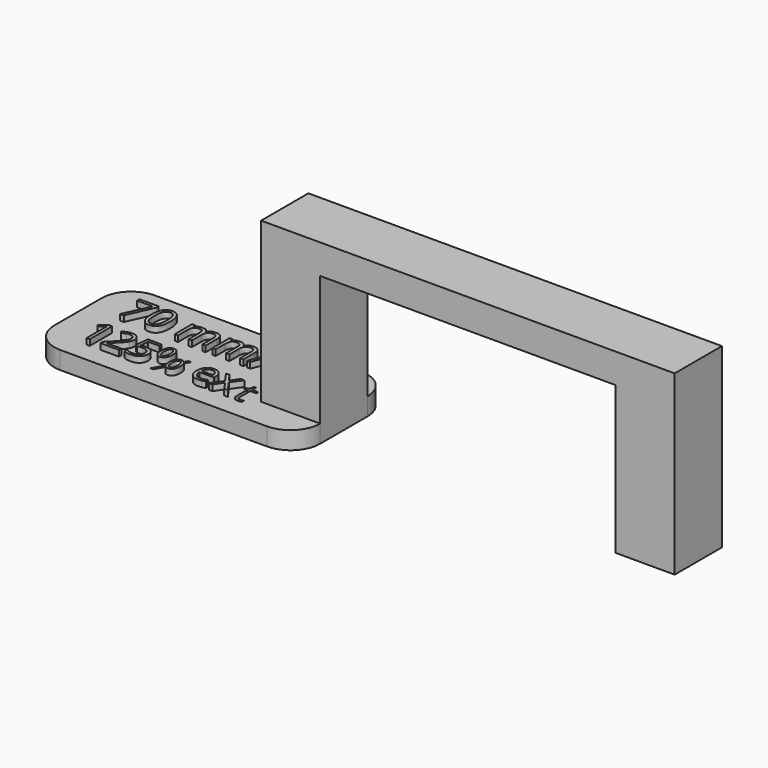
from build123d import *

# Parameters (mm, degrees)
F0_W         = 10
F0_H         = 10
F1_DEPTH     = 25
F2_START     = 25
F0_W_2       = 50
F2_DEPTH     = 5
F0_TEXT_SIZE = 6.8483603532
F3_DEPTH     = 3
F4_DEPTH     = 4


# Not quite as in the source:
# - Text() gives the source's letters only with a copy of the font that has no kerning and outlines rounded to 1/6400 em; it was checked with that copy


with BuildPart() as f1:
    # F0 (on Top) → F1 (new body)
    with BuildSketch(Plane.XY):
        with Locations((30, 0)):
            Rectangle(F0_W, F0_H)
    extrude(amount=F1_DEPTH)



with BuildPart() as f1b:
    # F0 (on Top) → F1, piece 2 (new body)
    with BuildSketch(Plane.XY):
        with Locations((-30, 0)):
            Rectangle(F0_W, F0_H)
    extrude(amount=F1_DEPTH)


with BuildPart() as f1_1:
    add(f1.part)

    add(f1b.part)  # F2 merges F1b
    # F0 (on Top) → F2 (join)
    with BuildSketch(Plane.XY.offset(F2_START)):
        Rectangle(F0_W_2, F0_H)
        with Locations((-30, 0)):
            Rectangle(F0_W, F0_H)
        with Locations((30, 0)):
            Rectangle(F0_W, F0_H)
    extrude(amount=F2_DEPTH)

    # F0 (on Top) → F3 (join)
    with BuildSketch(Plane.XY):
        with BuildLine():
            ThreePointArc((-30, -10), (-26.4644660941, -8.5355339059), (-25, -5))
            Line((-25, -5), (-35, -5))
            Line((-35, -5), (-35, 5))
            Line((-35, 5), (-25, 5))
            ThreePointArc((-25, 5), (-26.4644660941, 8.5355339059), (-30, 10))
            Line((-30, 10), (-65, 10))
            ThreePointArc((-65, 10), (-68.5355339059, 8.5355339059), (-70, 5))
            Line((-70, 5), (-70, -5))
            ThreePointArc((-70, -5), (-68.5355339059, -8.5355339059), (-65, -10))
            Line((-65, -10), (-30, -10))
        make_face()
        with BuildLine():
            add(Edge.make_bspline(
                [(-48.7220816963, -4.113544751), (-48.4639328914, -4.4947946962), (-48.4639328914, -5.2157414592)],
                knots=[0, 0, 0, 1, 1, 1], degree=2))
            add(Edge.make_bspline(
                [(-48.4639328914, -5.2157414592), (-48.4639328914, -5.9522706451), (-48.7122128285, -6.3309235199)],
                knots=[0, 0, 0, 1, 1, 1], degree=2))
            add(Edge.make_bspline(
                [(-48.7122128285, -6.3309235199), (-48.9604927656, -6.7095763947), (-49.441470217, -6.7095763947)],
                knots=[0, 0, 0, 1, 1, 1], degree=2))
            add(Edge.make_bspline(
                [(-49.441470217, -6.7095763947), (-49.9027099328, -6.7095763947), (-50.1509898699, -6.3231323084)],
                knots=[0, 0, 0, 1, 1, 1], degree=2))
            add(Edge.make_bspline(
                [(-50.1509898699, -6.3231323084), (-50.399269807, -5.9366882222), (-50.399269807, -5.2157414592)],
                knots=[0, 0, 0, 1, 1, 1], degree=2))
            add(Edge.make_bspline(
                [(-50.399269807, -5.2157414592), (-50.399269807, -4.4792122734), (-50.157222839, -4.1057535395)],
                knots=[0, 0, 0, 1, 1, 1], degree=2))
            add(Edge.make_bspline(
                [(-50.157222839, -4.1057535395), (-49.9151758711, -3.7322948057), (-49.441470217, -3.7322948057)],
                knots=[0, 0, 0, 1, 1, 1], degree=2))
            add(Edge.make_bspline(
                [(-49.441470217, -3.7322948057), (-48.9802305012, -3.7322948057), (-48.7220816963, -4.113544751)],
                knots=[0, 0, 0, 1, 1, 1], degree=2))
        make_face(mode=Mode.SUBTRACT)
        with BuildLine():
            Line((-62.6792578263, -1.8977242243), (-62.6792578263, -6.6441302188))
            Line((-62.6792578263, -6.6441302188), (-63.2049048898, -6.6441302188))
            Line((-63.2049048898, -6.6441302188), (-63.2049048898, -3.2617056362))
            add(Edge.make_bspline(
                [(-63.2049048898, -3.2617056362), (-63.2049048898, -2.8389025634), (-63.1789341851, -2.462846759)],
                knots=[0, 0, 0, 1, 1, 1], degree=2))
            add(Edge.make_bspline(
                [(-63.1789341851, -2.462846759), (-63.2464580174, -2.5314094195), (-63.3311225148, -2.605685635)],
                knots=[0, 0, 0, 1, 1, 1], degree=2))
            add(Edge.make_bspline(
                [(-63.3311225148, -2.605685635), (-63.4157870121, -2.6799618505), (-64.1034912731, -3.238851416)],
                knots=[0, 0, 0, 1, 1, 1], degree=2))
            Line((-64.1034912731, -3.238851416), (-64.389169025, -2.8690285808))
            Line((-64.389169025, -2.8690285808), (-63.1332257448, -1.8977242243))
            Line((-63.1332257448, -1.8977242243), (-62.6792578263, -1.8977242243))
        make_face(mode=Mode.SUBTRACT)
        with BuildLine():
            Line((-57.7541733834, -6.14445386), (-57.7541733834, -6.6441302188))
            Line((-57.7541733834, -6.6441302188), (-60.8737744343, -6.6441302188))
            Line((-60.8737744343, -6.6441302188), (-60.8737744343, -6.1797740184))
            Line((-60.8737744343, -6.1797740184), (-59.6240641232, -4.9238307382))
            add(Edge.make_bspline(
                [(-59.6240641232, -4.9238307382), (-59.0527086194, -4.3452034371), (-58.8709136863, -4.0984817422)],
                knots=[0, 0, 0, 1, 1, 1], degree=2))
            add(Edge.make_bspline(
                [(-58.8709136863, -4.0984817422), (-58.6891187533, -3.8517600474), (-58.5982212868, -3.6180237049)],
                knots=[0, 0, 0, 1, 1, 1], degree=2))
            add(Edge.make_bspline(
                [(-58.5982212868, -3.6180237049), (-58.5073238203, -3.3842873625), (-58.5073238203, -3.1152308616)],
                knots=[0, 0, 0, 1, 1, 1], degree=2))
            add(Edge.make_bspline(
                [(-58.5073238203, -3.1152308616), (-58.5073238203, -2.7350197445), (-58.7379436782, -2.5127105121)],
                knots=[0, 0, 0, 1, 1, 1], degree=2))
            add(Edge.make_bspline(
                [(-58.7379436782, -2.5127105121), (-58.9685635361, -2.2904012797), (-59.3778618424, -2.2904012797)],
                knots=[0, 0, 0, 1, 1, 1], degree=2))
            add(Edge.make_bspline(
                [(-59.3778618424, -2.2904012797), (-59.6728890481, -2.2904012797), (-59.9377902362, -2.3880511294)],
                knots=[0, 0, 0, 1, 1, 1], degree=2))
            add(Edge.make_bspline(
                [(-59.9377902362, -2.3880511294), (-60.2026914243, -2.4857009792), (-60.5268058192, -2.7422915418)],
                knots=[0, 0, 0, 1, 1, 1], degree=2))
            Line((-60.5268058192, -2.7422915418), (-60.8124835711, -2.3755851912))
            add(Edge.make_bspline(
                [(-60.8124835711, -2.3755851912), (-60.156982984, -1.8302003921), (-59.3840948116, -1.8302003921)],
                knots=[0, 0, 0, 1, 1, 1], degree=2))
            add(Edge.make_bspline(
                [(-59.3840948116, -1.8302003921), (-58.715089458, -1.8302003921), (-58.335397755, -2.1724942803)],
                knots=[0, 0, 0, 1, 1, 1], degree=2))
            add(Edge.make_bspline(
                [(-58.335397755, -2.1724942803), (-57.955706052, -2.5147881685), (-57.955706052, -3.0923766414)],
                knots=[0, 0, 0, 1, 1, 1], degree=2))
            add(Edge.make_bspline(
                [(-57.955706052, -3.0923766414), (-57.955706052, -3.5442669035), (-58.2091801301, -3.9857688837)],
                knots=[0, 0, 0, 1, 1, 1], degree=2))
            add(Edge.make_bspline(
                [(-58.2091801301, -3.9857688837), (-58.4626542082, -4.427270864), (-59.1565914382, -5.1025091867)],
                knots=[0, 0, 0, 1, 1, 1], degree=2))
            Line((-59.1565914382, -5.1025091867), (-60.195419627, -6.1184831553))
            Line((-60.195419627, -6.1184831553), (-60.195419627, -6.14445386))
            Line((-60.195419627, -6.14445386), (-57.7541733834, -6.14445386))
        make_face(mode=Mode.SUBTRACT)
        with BuildLine():
            add(Edge.make_bspline(
                [(-56.3330564212, -3.8195563735), (-55.9601171014, -3.744760744), (-55.5892554381, -3.744760744)],
                knots=[0, 0, 0, 1, 1, 1], degree=2))
            add(Edge.make_bspline(
                [(-55.5892554381, -3.744760744), (-54.8392214858, -3.744760744), (-54.4091466156, -4.1166612355)],
                knots=[0, 0, 0, 1, 1, 1], degree=2))
            add(Edge.make_bspline(
                [(-54.4091466156, -4.1166612355), (-53.9790717455, -4.4885617271), (-53.9790717455, -5.1347128605)],
                knots=[0, 0, 0, 1, 1, 1], degree=2))
            add(Edge.make_bspline(
                [(-53.9790717455, -5.1347128605), (-53.9790717455, -5.8712420463), (-54.4481026727, -6.2904092205)],
                knots=[0, 0, 0, 1, 1, 1], degree=2))
            add(Edge.make_bspline(
                [(-54.4481026727, -6.2904092205), (-54.9171335999, -6.7095763947), (-55.7419631818, -6.7095763947)],
                knots=[0, 0, 0, 1, 1, 1], degree=2))
            add(Edge.make_bspline(
                [(-55.7419631818, -6.7095763947), (-56.5439385435, -6.7095763947), (-56.9657027882, -6.452985832)],
                knots=[0, 0, 0, 1, 1, 1], degree=2))
            Line((-56.9657027882, -6.452985832), (-56.9657027882, -5.9335717377))
            add(Edge.make_bspline(
                [(-56.9657027882, -5.9335717377), (-56.739238243, -6.0790076841), (-56.4016190817, -6.1621139392)],
                knots=[0, 0, 0, 1, 1, 1], degree=2))
            add(Edge.make_bspline(
                [(-56.4016190817, -6.1621139392), (-56.0639999203, -6.2452201943), (-55.7357302127, -6.2452201943)],
                knots=[0, 0, 0, 1, 1, 1], degree=2))
            add(Edge.make_bspline(
                [(-55.7357302127, -6.2452201943), (-55.1643747089, -6.2452201943), (-54.8480515254, -5.9756442793)],
                knots=[0, 0, 0, 1, 1, 1], degree=2))
            add(Edge.make_bspline(
                [(-54.8480515254, -5.9756442793), (-54.5317283419, -5.7060683643), (-54.5317283419, -5.1960037236)],
                knots=[0, 0, 0, 1, 1, 1], degree=2))
            add(Edge.make_bspline(
                [(-54.5317283419, -5.1960037236), (-54.5317283419, -4.2028839752), (-55.7481961509, -4.2028839752)],
                knots=[0, 0, 0, 1, 1, 1], degree=2))
            add(Edge.make_bspline(
                [(-55.7481961509, -4.2028839752), (-56.056728123, -4.2028839752), (-56.5730257328, -4.2974173404)],
                knots=[0, 0, 0, 1, 1, 1], degree=2))
            Line((-56.5730257328, -4.2974173404), (-56.8524705156, -4.1187388919))
            Line((-56.8524705156, -4.1187388919), (-56.6737920671, -1.8977242243))
            Line((-56.6737920671, -1.8977242243), (-54.3135744223, -1.8977242243))
            Line((-54.3135744223, -1.8977242243), (-54.3135744223, -2.3942840986))
            Line((-54.3135744223, -2.3942840986), (-56.2125523513, -2.3942840986))
            Line((-56.2125523513, -2.3942840986), (-56.3330564212, -3.8195563735))
        make_face(mode=Mode.SUBTRACT)
        Polygon((-49.7790893783, -1.8977242243), (-49.3022672397, -1.8977242243), (-51.93465787, -6.6441302188), (-52.4114800086, -6.6441302188), align=None, mode=Mode.SUBTRACT)
        with BuildLine():
            add(Edge.make_bspline(
                [(-43.7060997869, -6.6555573289), (-43.9606126931, -6.7095763947), (-44.3210860746, -6.7095763947)],
                knots=[0, 0, 0, 1, 1, 1], degree=2))
            add(Edge.make_bspline(
                [(-44.3210860746, -6.7095763947), (-45.1095566699, -6.7095763947), (-45.5661216588, -6.2285989433)],
                knots=[0, 0, 0, 1, 1, 1], degree=2))
            add(Edge.make_bspline(
                [(-45.5661216588, -6.2285989433), (-46.0226866478, -5.7476214919), (-46.0226866478, -4.8947435489)],
                knots=[0, 0, 0, 1, 1, 1], degree=2))
            add(Edge.make_bspline(
                [(-46.0226866478, -4.8947435489), (-46.0226866478, -4.0335549804), (-45.5988447468, -3.5271262384)],
                knots=[0, 0, 0, 1, 1, 1], degree=2))
            add(Edge.make_bspline(
                [(-45.5988447468, -3.5271262384), (-45.1750028458, -3.0206974964), (-44.4602890519, -3.0206974964)],
                knots=[0, 0, 0, 1, 1, 1], degree=2))
            add(Edge.make_bspline(
                [(-44.4602890519, -3.0206974964), (-43.7923225265, -3.0206974964), (-43.4027619557, -3.4606412343)],
                knots=[0, 0, 0, 1, 1, 1], degree=2))
            add(Edge.make_bspline(
                [(-43.4027619557, -3.4606412343), (-43.013201385, -3.9005849723), (-43.013201385, -4.6215317353)],
                knots=[0, 0, 0, 1, 1, 1], degree=2))
            Line((-43.013201385, -4.6215317353), (-43.013201385, -4.9622673812))
            Line((-43.013201385, -4.9622673812), (-45.4637970822, -4.9622673812))
            add(Edge.make_bspline(
                [(-45.4637970822, -4.9622673812), (-45.4471758312, -5.588680779), (-45.1469544847, -5.913314588)],
                knots=[0, 0, 0, 1, 1, 1], degree=2))
            add(Edge.make_bspline(
                [(-45.1469544847, -5.913314588), (-44.8467331381, -6.237948397), (-44.301348339, -6.237948397)],
                knots=[0, 0, 0, 1, 1, 1], degree=2))
            add(Edge.make_bspline(
                [(-44.301348339, -6.237948397), (-43.7268763506, -6.237948397), (-43.1659091287, -5.9979790854)],
                knots=[0, 0, 0, 1, 1, 1], degree=2))
            Line((-43.1659091287, -5.9979790854), (-43.1659091287, -6.4789565368))
            add(Edge.make_bspline(
                [(-43.1659091287, -6.4789565368), (-43.4515868806, -6.601538263), (-43.7060997869, -6.6555573289)],
                knots=[0, 0, 0, 1, 1, 1], degree=2))
        make_face(mode=Mode.SUBTRACT)
        with BuildLine():
            add(Edge.make_bspline(
                [(-51.5773009731, -2.2161250642), (-51.323826895, -2.6020497363), (-51.323826895, -3.3136470456)],
                knots=[0, 0, 0, 1, 1, 1], degree=2))
            add(Edge.make_bspline(
                [(-51.323826895, -3.3136470456), (-51.323826895, -4.053292716), (-51.5726262462, -4.4314261767)],
                knots=[0, 0, 0, 1, 1, 1], degree=2))
            add(Edge.make_bspline(
                [(-51.5726262462, -4.4314261767), (-51.8214255974, -4.8095596374), (-52.3013642206, -4.8095596374)],
                knots=[0, 0, 0, 1, 1, 1], degree=2))
            add(Edge.make_bspline(
                [(-52.3013642206, -4.8095596374), (-52.7563709673, -4.8095596374), (-53.007767389, -4.4236349653)],
                knots=[0, 0, 0, 1, 1, 1], degree=2))
            add(Edge.make_bspline(
                [(-53.007767389, -4.4236349653), (-53.2591638107, -4.0377102932), (-53.2591638107, -3.3136470456)],
                knots=[0, 0, 0, 1, 1, 1], degree=2))
            add(Edge.make_bspline(
                [(-53.2591638107, -3.3136470456), (-53.2591638107, -2.5760790316), (-53.0171168427, -2.2031397118)],
                knots=[0, 0, 0, 1, 1, 1], degree=2))
            add(Edge.make_bspline(
                [(-53.0171168427, -2.2031397118), (-52.7750698747, -1.8302003921), (-52.3013642206, -1.8302003921)],
                knots=[0, 0, 0, 1, 1, 1], degree=2))
            add(Edge.make_bspline(
                [(-52.3013642206, -1.8302003921), (-51.8307750511, -1.8302003921), (-51.5773009731, -2.2161250642)],
                knots=[0, 0, 0, 1, 1, 1], degree=2))
        make_face(mode=Mode.SUBTRACT)
        Polygon((-42.5384569027, -6.6441302188), (-41.2368051822, -4.8230644039), (-42.474049555, -3.0861436723), (-41.8601020954, -3.0861436723), (-40.922040241, -4.4490862559), (-39.9870948711, -3.0861436723), (-39.3793803807, -3.0861436723), (-40.6166247535, -4.8230644039), (-39.314973033, -6.6441302188), (-39.9247651798, -6.6441302188), (-40.922040241, -5.2022366928), (-41.9286647559, -6.6441302188), align=None, mode=Mode.SUBTRACT)
        with BuildLine():
            add(Edge.make_bspline(
                [(-37.8803513043, -6.0919930364), (-37.7276435606, -6.2639191017), (-37.4617035442, -6.2639191017)],
                knots=[0, 0, 0, 1, 1, 1], degree=2))
            add(Edge.make_bspline(
                [(-37.4617035442, -6.2639191017), (-37.3183452542, -6.2639191017), (-37.185375246, -6.2431425379)],
                knots=[0, 0, 0, 1, 1, 1], degree=2))
            add(Edge.make_bspline(
                [(-37.185375246, -6.2431425379), (-37.0524052379, -6.2223659741), (-36.9744931237, -6.199511754)],
                knots=[0, 0, 0, 1, 1, 1], degree=2))
            Line((-36.9744931237, -6.199511754), (-36.9744931237, -6.6119265449))
            add(Edge.make_bspline(
                [(-36.9744931237, -6.6119265449), (-37.0617546916, -6.6534796725), (-37.2321225145, -6.6815280336)],
                knots=[0, 0, 0, 1, 1, 1], degree=2))
            add(Edge.make_bspline(
                [(-37.2321225145, -6.6815280336), (-37.4024903375, -6.7095763947), (-37.5396156584, -6.7095763947)],
                knots=[0, 0, 0, 1, 1, 1], degree=2))
            add(Edge.make_bspline(
                [(-37.5396156584, -6.7095763947), (-38.5711720498, -6.7095763947), (-38.5711720498, -5.621923281)],
                knots=[0, 0, 0, 1, 1, 1], degree=2))
            Line((-38.5711720498, -5.621923281), (-38.5711720498, -3.5047914324))
            Line((-38.5711720498, -3.5047914324), (-39.0812366905, -3.5047914324))
            Line((-39.0812366905, -3.5047914324), (-39.0812366905, -3.2450843852))
            Line((-39.0812366905, -3.2450843852), (-38.5711720498, -3.0206974964))
            Line((-38.5711720498, -3.0206974964), (-38.3447075047, -2.2613140904))
            Line((-38.3447075047, -2.2613140904), (-38.0330590481, -2.2613140904))
            Line((-38.0330590481, -2.2613140904), (-38.0330590481, -3.0861436723))
            Line((-38.0330590481, -3.0861436723), (-37.0004638284, -3.0861436723))
            Line((-37.0004638284, -3.0861436723), (-37.0004638284, -3.5047914324))
            Line((-37.0004638284, -3.5047914324), (-38.0330590481, -3.5047914324))
            Line((-38.0330590481, -3.5047914324), (-38.0330590481, -5.5990690609))
            add(Edge.make_bspline(
                [(-38.0330590481, -5.5990690609), (-38.0330590481, -5.9200669712), (-37.8803513043, -6.0919930364)],
                knots=[0, 0, 0, 1, 1, 1], degree=2))
        make_face(mode=Mode.SUBTRACT)
        Polygon((-63.4312974566, 1.4880931385), (-64.0465798321, 1.4880931385), (-62.0209632464, 5.865693483), (-64.6854034463, 5.865693483), (-64.6854034463, 6.3771803969), (-61.4324322785, 6.3771803969), (-61.4324322785, 5.9320369739), align=None, mode=Mode.SUBTRACT)
        with BuildLine():
            add(Edge.make_bspline(
                [(-57.9226475975, 5.8084454707), (-57.5096058637, 5.1626664905), (-57.5096058637, 3.9395921337)],
                knots=[0, 0, 0, 1, 1, 1], degree=2))
            add(Edge.make_bspline(
                [(-57.5096058637, 3.9395921337), (-57.5096058637, 2.671575412), (-57.9092718937, 2.0461275016)],
                knots=[0, 0, 0, 1, 1, 1], degree=2))
            add(Edge.make_bspline(
                [(-57.9092718937, 2.0461275016), (-58.3089379237, 1.4206795913), (-59.1318112224, 1.4206795913)],
                knots=[0, 0, 0, 1, 1, 1], degree=2))
            add(Edge.make_bspline(
                [(-59.1318112224, 1.4206795913), (-59.9204427193, 1.4206795913), (-60.3318793686, 2.0611082899)],
                knots=[0, 0, 0, 1, 1, 1], degree=2))
            add(Edge.make_bspline(
                [(-60.3318793686, 2.0611082899), (-60.743316018, 2.7015369886), (-60.743316018, 3.9395921337)],
                knots=[0, 0, 0, 1, 1, 1], degree=2))
            add(Edge.make_bspline(
                [(-60.743316018, 3.9395921337), (-60.743316018, 5.2161693058), (-60.3452550724, 5.8351968783)],
                knots=[0, 0, 0, 1, 1, 1], degree=2))
            add(Edge.make_bspline(
                [(-60.3452550724, 5.8351968783), (-59.9471941269, 6.4542244509), (-59.1318112224, 6.4542244509)],
                knots=[0, 0, 0, 1, 1, 1], degree=2))
            add(Edge.make_bspline(
                [(-59.1318112224, 6.4542244509), (-58.3356893313, 6.4542244509), (-57.9226475975, 5.8084454707)],
                knots=[0, 0, 0, 1, 1, 1], degree=2))
        make_face(mode=Mode.SUBTRACT)
        with BuildLine():
            Line((-49.5751383607, 1.4880931385), (-50.1294275268, 1.4880931385))
            Line((-50.1294275268, 1.4880931385), (-50.1294275268, 3.8721785864))
            add(Edge.make_bspline(
                [(-50.1294275268, 3.8721785864), (-50.1294275268, 4.3109016716), (-50.3166873802, 4.529728186)],
                knots=[0, 0, 0, 1, 1, 1], degree=2))
            add(Edge.make_bspline(
                [(-50.3166873802, 4.529728186), (-50.5039472336, 4.7485547004), (-50.8987980103, 4.7485547004)],
                knots=[0, 0, 0, 1, 1, 1], degree=2))
            add(Edge.make_bspline(
                [(-50.8987980103, 4.7485547004), (-51.416705262, 4.7485547004), (-51.6644232966, 4.4510790475)],
                knots=[0, 0, 0, 1, 1, 1], degree=2))
            add(Edge.make_bspline(
                [(-51.6644232966, 4.4510790475), (-51.9121413313, 4.1536033947), (-51.9121413313, 3.5351108503)],
                knots=[0, 0, 0, 1, 1, 1], degree=2))
            Line((-51.9121413313, 3.5351108503), (-51.9121413313, 1.4880931385))
            Line((-51.9121413313, 1.4880931385), (-52.4675005537, 1.4880931385))
            Line((-52.4675005537, 1.4880931385), (-52.4675005537, 3.8721785864))
            add(Edge.make_bspline(
                [(-52.4675005537, 3.8721785864), (-52.4675005537, 4.3109016716), (-52.6547604071, 4.529728186)],
                knots=[0, 0, 0, 1, 1, 1], degree=2))
            add(Edge.make_bspline(
                [(-52.6547604071, 4.529728186), (-52.8420202605, 4.7485547004), (-53.240081206, 4.7485547004)],
                knots=[0, 0, 0, 1, 1, 1], degree=2))
            add(Edge.make_bspline(
                [(-53.240081206, 4.7485547004), (-53.7611986266, 4.7485547004), (-54.0035663797, 4.4360982593)],
                knots=[0, 0, 0, 1, 1, 1], degree=2))
            add(Edge.make_bspline(
                [(-54.0035663797, 4.4360982593), (-54.2459341329, 4.1236418182), (-54.2459341329, 3.4109843189)],
                knots=[0, 0, 0, 1, 1, 1], degree=2))
            Line((-54.2459341329, 3.4109843189), (-54.2459341329, 1.4880931385))
            Line((-54.2459341329, 1.4880931385), (-54.8012933553, 1.4880931385))
            Line((-54.8012933553, 1.4880931385), (-54.8012933553, 5.1530359837))
            Line((-54.8012933553, 5.1530359837), (-54.3497295945, 5.1530359837))
            Line((-54.3497295945, 5.1530359837), (-54.2598448648, 4.6511795766))
            Line((-54.2598448648, 4.6511795766), (-54.2330934572, 4.6511795766))
            add(Edge.make_bspline(
                [(-54.2330934572, 4.6511795766), (-54.0757951803, 4.9186936529), (-53.7895551187, 5.0695715919)],
                knots=[0, 0, 0, 1, 1, 1], degree=2))
            add(Edge.make_bspline(
                [(-53.7895551187, 5.0695715919), (-53.5033150571, 5.220449531), (-53.1491264201, 5.220449531)],
                knots=[0, 0, 0, 1, 1, 1], degree=2))
            add(Edge.make_bspline(
                [(-53.1491264201, 5.220449531), (-52.289871207, 5.220449531), (-52.0255672996, 4.5976767614)],
                knots=[0, 0, 0, 1, 1, 1], degree=2))
            Line((-52.0255672996, 4.5976767614), (-51.998815892, 4.5976767614))
            add(Edge.make_bspline(
                [(-51.998815892, 4.5976767614), (-51.8350972773, 4.8855219074), (-51.5242459206, 5.0529857192)],
                knots=[0, 0, 0, 1, 1, 1], degree=2))
            add(Edge.make_bspline(
                [(-51.5242459206, 5.0529857192), (-51.213394564, 5.220449531), (-50.8153336184, 5.220449531)],
                knots=[0, 0, 0, 1, 1, 1], degree=2))
            add(Edge.make_bspline(
                [(-50.8153336184, 5.220449531), (-50.1936309051, 5.220449531), (-49.8843846329, 4.9010377239)],
                knots=[0, 0, 0, 1, 1, 1], degree=2))
            add(Edge.make_bspline(
                [(-49.8843846329, 4.9010377239), (-49.5751383607, 4.5816259168), (-49.5751383607, 3.8785989243)],
                knots=[0, 0, 0, 1, 1, 1], degree=2))
            Line((-49.5751383607, 3.8785989243), (-49.5751383607, 1.4880931385))
        make_face(mode=Mode.SUBTRACT)
        with BuildLine():
            Line((-43.205093176, 1.4880931385), (-43.759382342, 1.4880931385))
            Line((-43.759382342, 1.4880931385), (-43.759382342, 3.8721785864))
            add(Edge.make_bspline(
                [(-43.759382342, 3.8721785864), (-43.759382342, 4.3109016716), (-43.9466421955, 4.529728186)],
                knots=[0, 0, 0, 1, 1, 1], degree=2))
            add(Edge.make_bspline(
                [(-43.9466421955, 4.529728186), (-44.1339020489, 4.7485547004), (-44.5287528255, 4.7485547004)],
                knots=[0, 0, 0, 1, 1, 1], degree=2))
            add(Edge.make_bspline(
                [(-44.5287528255, 4.7485547004), (-45.0466600772, 4.7485547004), (-45.2943781118, 4.4510790475)],
                knots=[0, 0, 0, 1, 1, 1], degree=2))
            add(Edge.make_bspline(
                [(-45.2943781118, 4.4510790475), (-45.5420961465, 4.1536033947), (-45.5420961465, 3.5351108503)],
                knots=[0, 0, 0, 1, 1, 1], degree=2))
            Line((-45.5420961465, 3.5351108503), (-45.5420961465, 1.4880931385))
            Line((-45.5420961465, 1.4880931385), (-46.0974553689, 1.4880931385))
            Line((-46.0974553689, 1.4880931385), (-46.0974553689, 3.8721785864))
            add(Edge.make_bspline(
                [(-46.0974553689, 3.8721785864), (-46.0974553689, 4.3109016716), (-46.2847152223, 4.529728186)],
                knots=[0, 0, 0, 1, 1, 1], degree=2))
            add(Edge.make_bspline(
                [(-46.2847152223, 4.529728186), (-46.4719750757, 4.7485547004), (-46.8700360212, 4.7485547004)],
                knots=[0, 0, 0, 1, 1, 1], degree=2))
            add(Edge.make_bspline(
                [(-46.8700360212, 4.7485547004), (-47.3911534418, 4.7485547004), (-47.633521195, 4.4360982593)],
                knots=[0, 0, 0, 1, 1, 1], degree=2))
            add(Edge.make_bspline(
                [(-47.633521195, 4.4360982593), (-47.8758889481, 4.1236418182), (-47.8758889481, 3.4109843189)],
                knots=[0, 0, 0, 1, 1, 1], degree=2))
            Line((-47.8758889481, 3.4109843189), (-47.8758889481, 1.4880931385))
            Line((-47.8758889481, 1.4880931385), (-48.4312481705, 1.4880931385))
            Line((-48.4312481705, 1.4880931385), (-48.4312481705, 5.1530359837))
            Line((-48.4312481705, 5.1530359837), (-47.9796844097, 5.1530359837))
            Line((-47.9796844097, 5.1530359837), (-47.8897996801, 4.6511795766))
            Line((-47.8897996801, 4.6511795766), (-47.8630482724, 4.6511795766))
            add(Edge.make_bspline(
                [(-47.8630482724, 4.6511795766), (-47.7057499956, 4.9186936529), (-47.4195099339, 5.0695715919)],
                knots=[0, 0, 0, 1, 1, 1], degree=2))
            add(Edge.make_bspline(
                [(-47.4195099339, 5.0695715919), (-47.1332698723, 5.220449531), (-46.7790812353, 5.220449531)],
                knots=[0, 0, 0, 1, 1, 1], degree=2))
            add(Edge.make_bspline(
                [(-46.7790812353, 5.220449531), (-45.9198260222, 5.220449531), (-45.6555221148, 4.5976767614)],
                knots=[0, 0, 0, 1, 1, 1], degree=2))
            Line((-45.6555221148, 4.5976767614), (-45.6287707072, 4.5976767614))
            add(Edge.make_bspline(
                [(-45.6287707072, 4.5976767614), (-45.4650520925, 4.8855219074), (-45.1542007359, 5.0529857192)],
                knots=[0, 0, 0, 1, 1, 1], degree=2))
            add(Edge.make_bspline(
                [(-45.1542007359, 5.0529857192), (-44.8433493792, 5.220449531), (-44.4452884337, 5.220449531)],
                knots=[0, 0, 0, 1, 1, 1], degree=2))
            add(Edge.make_bspline(
                [(-44.4452884337, 5.220449531), (-43.8235857204, 5.220449531), (-43.5143394482, 4.9010377239)],
                knots=[0, 0, 0, 1, 1, 1], degree=2))
            add(Edge.make_bspline(
                [(-43.5143394482, 4.9010377239), (-43.205093176, 4.5816259168), (-43.205093176, 3.8785989243)],
                knots=[0, 0, 0, 1, 1, 1], degree=2))
            Line((-43.205093176, 3.8785989243), (-43.205093176, 1.4880931385))
        make_face(mode=Mode.SUBTRACT)
        with BuildLine():
            add(Edge.make_bspline(
                [(-37.4118083397, 3.0931775963), (-37.1828162904, 2.8524149276), (-37.1828162904, 2.4875257275)],
                knots=[0, 0, 0, 1, 1, 1], degree=2))
            add(Edge.make_bspline(
                [(-37.1828162904, 2.4875257275), (-37.1828162904, 1.9760388136), (-37.563756335, 1.6983592025)],
                knots=[0, 0, 0, 1, 1, 1], degree=2))
            add(Edge.make_bspline(
                [(-37.563756335, 1.6983592025), (-37.9446963797, 1.4206795913), (-38.6338126402, 1.4206795913)],
                knots=[0, 0, 0, 1, 1, 1], degree=2))
            add(Edge.make_bspline(
                [(-38.6338126402, 1.4206795913), (-39.362520984, 1.4206795913), (-39.7702124363, 1.6518117532)],
                knots=[0, 0, 0, 1, 1, 1], degree=2))
            Line((-39.7702124363, 1.6518117532), (-39.7702124363, 2.166508836))
            add(Edge.make_bspline(
                [(-39.7702124363, 2.166508836), (-39.5059085289, 2.0327517978), (-39.2036176227, 1.956242772)],
                knots=[0, 0, 0, 1, 1, 1], degree=2))
            add(Edge.make_bspline(
                [(-39.2036176227, 1.956242772), (-38.9013267165, 1.8797337462), (-38.6199019082, 1.8797337462)],
                knots=[0, 0, 0, 1, 1, 1], degree=2))
            add(Edge.make_bspline(
                [(-38.6199019082, 1.8797337462), (-38.1854590483, 1.8797337462), (-37.9516517456, 2.0183060377)],
                knots=[0, 0, 0, 1, 1, 1], degree=2))
            add(Edge.make_bspline(
                [(-37.9516517456, 2.0183060377), (-37.717844443, 2.1568783292), (-37.717844443, 2.4415133064)],
                knots=[0, 0, 0, 1, 1, 1], degree=2))
            add(Edge.make_bspline(
                [(-37.717844443, 2.4415133064), (-37.717844443, 2.6555245674), (-37.9029641838, 2.8074725628)],
                knots=[0, 0, 0, 1, 1, 1], degree=2))
            add(Edge.make_bspline(
                [(-37.9029641838, 2.8074725628), (-38.0880839246, 2.9594205581), (-38.6273923024, 3.1670114813)],
                knots=[0, 0, 0, 1, 1, 1], degree=2))
            add(Edge.make_bspline(
                [(-38.6273923024, 3.1670114813), (-39.1388792162, 3.3574815036), (-39.3544955617, 3.4997989922)],
                knots=[0, 0, 0, 1, 1, 1], degree=2))
            add(Edge.make_bspline(
                [(-39.3544955617, 3.4997989922), (-39.5701119072, 3.6421164808), (-39.6755124533, 3.8224209682)],
                knots=[0, 0, 0, 1, 1, 1], degree=2))
            add(Edge.make_bspline(
                [(-39.6755124533, 3.8224209682), (-39.7809129994, 4.0027254557), (-39.7809129994, 4.2531186311)],
                knots=[0, 0, 0, 1, 1, 1], degree=2))
            add(Edge.make_bspline(
                [(-39.7809129994, 4.2531186311), (-39.7809129994, 4.701472223), (-39.4160237993, 4.960960877)],
                knots=[0, 0, 0, 1, 1, 1], degree=2))
            add(Edge.make_bspline(
                [(-39.4160237993, 4.960960877), (-39.0511345992, 5.220449531), (-38.4165912102, 5.220449531)],
                knots=[0, 0, 0, 1, 1, 1], degree=2))
            add(Edge.make_bspline(
                [(-38.4165912102, 5.220449531), (-37.8248500735, 5.220449531), (-37.258790288, 4.9796868623)],
                knots=[0, 0, 0, 1, 1, 1], degree=2))
            Line((-37.258790288, 4.9796868623), (-37.4567507045, 4.5281231015))
            add(Edge.make_bspline(
                [(-37.4567507045, 4.5281231015), (-38.0078297017, 4.7549750382), (-38.4561832935, 4.7549750382)],
                knots=[0, 0, 0, 1, 1, 1], degree=2))
            add(Edge.make_bspline(
                [(-38.4561832935, 4.7549750382), (-38.8510340702, 4.7549750382), (-39.0516696274, 4.631383535)],
                knots=[0, 0, 0, 1, 1, 1], degree=2))
            add(Edge.make_bspline(
                [(-39.0516696274, 4.631383535), (-39.2523051846, 4.5077920317), (-39.2523051846, 4.2905706018)],
                knots=[0, 0, 0, 1, 1, 1], degree=2))
            add(Edge.make_bspline(
                [(-39.2523051846, 4.2905706018), (-39.2523051846, 4.1429028317), (-39.1768662151, 4.0396423982)],
                knots=[0, 0, 0, 1, 1, 1], degree=2))
            add(Edge.make_bspline(
                [(-39.1768662151, 4.0396423982), (-39.1014272456, 3.9363819647), (-38.934498462, 3.842752038)],
                knots=[0, 0, 0, 1, 1, 1], degree=2))
            add(Edge.make_bspline(
                [(-38.934498462, 3.842752038), (-38.7675696783, 3.7491221113), (-38.2924646788, 3.5714927647)],
                knots=[0, 0, 0, 1, 1, 1], degree=2))
            add(Edge.make_bspline(
                [(-38.2924646788, 3.5714927647), (-37.640800389, 3.3339402649), (-37.4118083397, 3.0931775963)],
                knots=[0, 0, 0, 1, 1, 1], degree=2))
        make_face(mode=Mode.SUBTRACT)
        Polygon((-40.7600145186, 6.3771803969), (-40.2057253525, 6.3771803969), (-42.0280312403, 1.4880931385), (-42.5823204063, 1.4880931385), align=None, mode=Mode.SUBTRACT)
        with Locations((-30, 0)):
            Rectangle(F0_W, F0_H)
        with BuildLine():
            add(Edge.make_bspline(
                [(-59.9306082542, 5.4895686917), (-60.1815364577, 5.0064382699), (-60.1815364577, 3.9395921337)],
                knots=[0, 0, 0, 1, 1, 1], degree=2))
            add(Edge.make_bspline(
                [(-60.1815364577, 3.9395921337), (-60.1815364577, 2.8727459974), (-59.9306082542, 2.3858703785)],
                knots=[0, 0, 0, 1, 1, 1], degree=2))
            add(Edge.make_bspline(
                [(-59.9306082542, 2.3858703785), (-59.6796800506, 1.8989947597), (-59.1318112224, 1.8989947597)],
                knots=[0, 0, 0, 1, 1, 1], degree=2))
            add(Edge.make_bspline(
                [(-59.1318112224, 1.8989947597), (-58.576452, 1.8989947597), (-58.327663909, 2.3922907164)],
                knots=[0, 0, 0, 1, 1, 1], degree=2))
            add(Edge.make_bspline(
                [(-58.327663909, 2.3922907164), (-58.0788758181, 2.8855866731), (-58.0788758181, 3.9395921337)],
                knots=[0, 0, 0, 1, 1, 1], degree=2))
            add(Edge.make_bspline(
                [(-58.0788758181, 3.9395921337), (-58.0788758181, 4.992527538), (-58.327663909, 5.4826133257)],
                knots=[0, 0, 0, 1, 1, 1], degree=2))
            add(Edge.make_bspline(
                [(-58.327663909, 5.4826133257), (-58.576452, 5.9726991135), (-59.1318112224, 5.9726991135)],
                knots=[0, 0, 0, 1, 1, 1], degree=2))
            add(Edge.make_bspline(
                [(-59.1318112224, 5.9726991135), (-59.6796800506, 5.9726991135), (-59.9306082542, 5.4895686917)],
                knots=[0, 0, 0, 1, 1, 1], degree=2))
        make_face()
        with BuildLine():
            add(Edge.make_bspline(
                [(-44.3210860746, -6.7095763947), (-45.1095566699, -6.7095763947), (-45.5661216588, -6.2285989433)],
                knots=[0, 0, 0, 1, 1, 1], degree=2))
            add(Edge.make_bspline(
                [(-43.7060997869, -6.6555573289), (-43.9606126931, -6.7095763947), (-44.3210860746, -6.7095763947)],
                knots=[0, 0, 0, 1, 1, 1], degree=2))
            add(Edge.make_bspline(
                [(-43.1659091287, -6.4789565368), (-43.4515868806, -6.601538263), (-43.7060997869, -6.6555573289)],
                knots=[0, 0, 0, 1, 1, 1], degree=2))
            Line((-43.1659091287, -6.4789565368), (-43.1659091287, -5.9979790854))
            add(Edge.make_bspline(
                [(-44.301348339, -6.237948397), (-43.7268763506, -6.237948397), (-43.1659091287, -5.9979790854)],
                knots=[0, 0, 0, 1, 1, 1], degree=2))
            add(Edge.make_bspline(
                [(-45.1469544847, -5.913314588), (-44.8467331381, -6.237948397), (-44.301348339, -6.237948397)],
                knots=[0, 0, 0, 1, 1, 1], degree=2))
            add(Edge.make_bspline(
                [(-45.4637970822, -4.9622673812), (-45.4471758312, -5.588680779), (-45.1469544847, -5.913314588)],
                knots=[0, 0, 0, 1, 1, 1], degree=2))
            Line((-45.4637970822, -4.9622673812), (-43.013201385, -4.9622673812))
            Line((-43.013201385, -4.9622673812), (-43.013201385, -4.6215317353))
            add(Edge.make_bspline(
                [(-43.4027619557, -3.4606412343), (-43.013201385, -3.9005849723), (-43.013201385, -4.6215317353)],
                knots=[0, 0, 0, 1, 1, 1], degree=2))
            add(Edge.make_bspline(
                [(-44.4602890519, -3.0206974964), (-43.7923225265, -3.0206974964), (-43.4027619557, -3.4606412343)],
                knots=[0, 0, 0, 1, 1, 1], degree=2))
            add(Edge.make_bspline(
                [(-45.5988447468, -3.5271262384), (-45.1750028458, -3.0206974964), (-44.4602890519, -3.0206974964)],
                knots=[0, 0, 0, 1, 1, 1], degree=2))
            add(Edge.make_bspline(
                [(-46.0226866478, -4.8947435489), (-46.0226866478, -4.0335549804), (-45.5988447468, -3.5271262384)],
                knots=[0, 0, 0, 1, 1, 1], degree=2))
            add(Edge.make_bspline(
                [(-45.5661216588, -6.2285989433), (-46.0226866478, -5.7476214919), (-46.0226866478, -4.8947435489)],
                knots=[0, 0, 0, 1, 1, 1], degree=2))
        make_face()
        with BuildLine():
            add(Edge.make_bspline(
                [(-44.4675608492, -3.4725877585), (-44.895558063, -3.4725877585), (-45.1505903833, -3.7515131272)],
                knots=[0, 0, 0, 1, 1, 1], degree=2))
            add(Edge.make_bspline(
                [(-43.8177738172, -3.7437219158), (-44.0447577764, -3.4725877585), (-44.4675608492, -3.4725877585)],
                knots=[0, 0, 0, 1, 1, 1], degree=2))
            add(Edge.make_bspline(
                [(-43.5907898579, -4.5238818855), (-43.5907898579, -4.014856073), (-43.8177738172, -3.7437219158)],
                knots=[0, 0, 0, 1, 1, 1], degree=2))
            Line((-43.5907898579, -4.5238818855), (-45.451331144, -4.5238818855))
            add(Edge.make_bspline(
                [(-45.1505903833, -3.7515131272), (-45.4056227037, -4.0304384959), (-45.451331144, -4.5238818855)],
                knots=[0, 0, 0, 1, 1, 1], degree=2))
        make_face(mode=Mode.SUBTRACT)
        with BuildLine():
            add(Edge.make_bspline(
                [(-55.5892554381, -3.744760744), (-54.8392214858, -3.744760744), (-54.4091466156, -4.1166612355)],
                knots=[0, 0, 0, 1, 1, 1], degree=2))
            add(Edge.make_bspline(
                [(-56.3330564212, -3.8195563735), (-55.9601171014, -3.744760744), (-55.5892554381, -3.744760744)],
                knots=[0, 0, 0, 1, 1, 1], degree=2))
            Line((-56.3330564212, -3.8195563735), (-56.2125523513, -2.3942840986))
            Line((-56.2125523513, -2.3942840986), (-54.3135744223, -2.3942840986))
            Line((-54.3135744223, -2.3942840986), (-54.3135744223, -1.8977242243))
            Line((-54.3135744223, -1.8977242243), (-56.6737920671, -1.8977242243))
            Line((-56.6737920671, -1.8977242243), (-56.8524705156, -4.1187388919))
            Line((-56.8524705156, -4.1187388919), (-56.5730257328, -4.2974173404))
            add(Edge.make_bspline(
                [(-55.7481961509, -4.2028839752), (-56.056728123, -4.2028839752), (-56.5730257328, -4.2974173404)],
                knots=[0, 0, 0, 1, 1, 1], degree=2))
            add(Edge.make_bspline(
                [(-54.5317283419, -5.1960037236), (-54.5317283419, -4.2028839752), (-55.7481961509, -4.2028839752)],
                knots=[0, 0, 0, 1, 1, 1], degree=2))
            add(Edge.make_bspline(
                [(-54.8480515254, -5.9756442793), (-54.5317283419, -5.7060683643), (-54.5317283419, -5.1960037236)],
                knots=[0, 0, 0, 1, 1, 1], degree=2))
            add(Edge.make_bspline(
                [(-55.7357302127, -6.2452201943), (-55.1643747089, -6.2452201943), (-54.8480515254, -5.9756442793)],
                knots=[0, 0, 0, 1, 1, 1], degree=2))
            add(Edge.make_bspline(
                [(-56.4016190817, -6.1621139392), (-56.0639999203, -6.2452201943), (-55.7357302127, -6.2452201943)],
                knots=[0, 0, 0, 1, 1, 1], degree=2))
            add(Edge.make_bspline(
                [(-56.9657027882, -5.9335717377), (-56.739238243, -6.0790076841), (-56.4016190817, -6.1621139392)],
                knots=[0, 0, 0, 1, 1, 1], degree=2))
            Line((-56.9657027882, -5.9335717377), (-56.9657027882, -6.452985832))
            add(Edge.make_bspline(
                [(-55.7419631818, -6.7095763947), (-56.5439385435, -6.7095763947), (-56.9657027882, -6.452985832)],
                knots=[0, 0, 0, 1, 1, 1], degree=2))
            add(Edge.make_bspline(
                [(-54.4481026727, -6.2904092205), (-54.9171335999, -6.7095763947), (-55.7419631818, -6.7095763947)],
                knots=[0, 0, 0, 1, 1, 1], degree=2))
            add(Edge.make_bspline(
                [(-53.9790717455, -5.1347128605), (-53.9790717455, -5.8712420463), (-54.4481026727, -6.2904092205)],
                knots=[0, 0, 0, 1, 1, 1], degree=2))
            add(Edge.make_bspline(
                [(-54.4091466156, -4.1166612355), (-53.9790717455, -4.4885617271), (-53.9790717455, -5.1347128605)],
                knots=[0, 0, 0, 1, 1, 1], degree=2))
        make_face()
        with BuildLine():
            Line((-60.8737744343, -6.6441302188), (-57.7541733834, -6.6441302188))
            Line((-57.7541733834, -6.6441302188), (-57.7541733834, -6.14445386))
            Line((-57.7541733834, -6.14445386), (-60.195419627, -6.14445386))
            Line((-60.195419627, -6.14445386), (-60.195419627, -6.1184831553))
            Line((-60.195419627, -6.1184831553), (-59.1565914382, -5.1025091867))
            add(Edge.make_bspline(
                [(-58.2091801301, -3.9857688837), (-58.4626542082, -4.427270864), (-59.1565914382, -5.1025091867)],
                knots=[0, 0, 0, 1, 1, 1], degree=2))
            add(Edge.make_bspline(
                [(-57.955706052, -3.0923766414), (-57.955706052, -3.5442669035), (-58.2091801301, -3.9857688837)],
                knots=[0, 0, 0, 1, 1, 1], degree=2))
            add(Edge.make_bspline(
                [(-58.335397755, -2.1724942803), (-57.955706052, -2.5147881685), (-57.955706052, -3.0923766414)],
                knots=[0, 0, 0, 1, 1, 1], degree=2))
            add(Edge.make_bspline(
                [(-59.3840948116, -1.8302003921), (-58.715089458, -1.8302003921), (-58.335397755, -2.1724942803)],
                knots=[0, 0, 0, 1, 1, 1], degree=2))
            add(Edge.make_bspline(
                [(-60.8124835711, -2.3755851912), (-60.156982984, -1.8302003921), (-59.3840948116, -1.8302003921)],
                knots=[0, 0, 0, 1, 1, 1], degree=2))
            Line((-60.8124835711, -2.3755851912), (-60.5268058192, -2.7422915418))
            add(Edge.make_bspline(
                [(-59.9377902362, -2.3880511294), (-60.2026914243, -2.4857009792), (-60.5268058192, -2.7422915418)],
                knots=[0, 0, 0, 1, 1, 1], degree=2))
            add(Edge.make_bspline(
                [(-59.3778618424, -2.2904012797), (-59.6728890481, -2.2904012797), (-59.9377902362, -2.3880511294)],
                knots=[0, 0, 0, 1, 1, 1], degree=2))
            add(Edge.make_bspline(
                [(-58.7379436782, -2.5127105121), (-58.9685635361, -2.2904012797), (-59.3778618424, -2.2904012797)],
                knots=[0, 0, 0, 1, 1, 1], degree=2))
            add(Edge.make_bspline(
                [(-58.5073238203, -3.1152308616), (-58.5073238203, -2.7350197445), (-58.7379436782, -2.5127105121)],
                knots=[0, 0, 0, 1, 1, 1], degree=2))
            add(Edge.make_bspline(
                [(-58.5982212868, -3.6180237049), (-58.5073238203, -3.3842873625), (-58.5073238203, -3.1152308616)],
                knots=[0, 0, 0, 1, 1, 1], degree=2))
            add(Edge.make_bspline(
                [(-58.8709136863, -4.0984817422), (-58.6891187533, -3.8517600474), (-58.5982212868, -3.6180237049)],
                knots=[0, 0, 0, 1, 1, 1], degree=2))
            add(Edge.make_bspline(
                [(-59.6240641232, -4.9238307382), (-59.0527086194, -4.3452034371), (-58.8709136863, -4.0984817422)],
                knots=[0, 0, 0, 1, 1, 1], degree=2))
            Line((-59.6240641232, -4.9238307382), (-60.8737744343, -6.1797740184))
            Line((-60.8737744343, -6.1797740184), (-60.8737744343, -6.6441302188))
        make_face()
        with BuildLine():
            add(Edge.make_bspline(
                [(-51.323826895, -3.3136470456), (-51.323826895, -4.053292716), (-51.5726262462, -4.4314261767)],
                knots=[0, 0, 0, 1, 1, 1], degree=2))
            add(Edge.make_bspline(
                [(-51.5773009731, -2.2161250642), (-51.323826895, -2.6020497363), (-51.323826895, -3.3136470456)],
                knots=[0, 0, 0, 1, 1, 1], degree=2))
            add(Edge.make_bspline(
                [(-52.3013642206, -1.8302003921), (-51.8307750511, -1.8302003921), (-51.5773009731, -2.2161250642)],
                knots=[0, 0, 0, 1, 1, 1], degree=2))
            add(Edge.make_bspline(
                [(-53.0171168427, -2.2031397118), (-52.7750698747, -1.8302003921), (-52.3013642206, -1.8302003921)],
                knots=[0, 0, 0, 1, 1, 1], degree=2))
            add(Edge.make_bspline(
                [(-53.2591638107, -3.3136470456), (-53.2591638107, -2.5760790316), (-53.0171168427, -2.2031397118)],
                knots=[0, 0, 0, 1, 1, 1], degree=2))
            add(Edge.make_bspline(
                [(-53.007767389, -4.4236349653), (-53.2591638107, -4.0377102932), (-53.2591638107, -3.3136470456)],
                knots=[0, 0, 0, 1, 1, 1], degree=2))
            add(Edge.make_bspline(
                [(-52.3013642206, -4.8095596374), (-52.7563709673, -4.8095596374), (-53.007767389, -4.4236349653)],
                knots=[0, 0, 0, 1, 1, 1], degree=2))
            add(Edge.make_bspline(
                [(-51.5726262462, -4.4314261767), (-51.8214255974, -4.8095596374), (-52.3013642206, -4.8095596374)],
                knots=[0, 0, 0, 1, 1, 1], degree=2))
        make_face()
        with BuildLine():
            add(Edge.make_bspline(
                [(-52.8114288613, -3.3136470456), (-52.8114288613, -3.8652648138), (-52.6909247914, -4.141073698)],
                knots=[0, 0, 0, 1, 1, 1], degree=2))
            add(Edge.make_bspline(
                [(-52.6909247914, -2.4882980497), (-52.8114288613, -2.7609904492), (-52.8114288613, -3.3136470456)],
                knots=[0, 0, 0, 1, 1, 1], degree=2))
            add(Edge.make_bspline(
                [(-52.3013642206, -2.2156056501), (-52.5704207215, -2.2156056501), (-52.6909247914, -2.4882980497)],
                knots=[0, 0, 0, 1, 1, 1], degree=2))
            add(Edge.make_bspline(
                [(-51.769484188, -3.3136470456), (-51.769484188, -2.2156056501), (-52.3013642206, -2.2156056501)],
                knots=[0, 0, 0, 1, 1, 1], degree=2))
            add(Edge.make_bspline(
                [(-52.3013642206, -4.4168825821), (-51.769484188, -4.4168825821), (-51.769484188, -3.3136470456)],
                knots=[0, 0, 0, 1, 1, 1], degree=2))
            add(Edge.make_bspline(
                [(-52.6909247914, -4.141073698), (-52.5704207215, -4.4168825821), (-52.3013642206, -4.4168825821)],
                knots=[0, 0, 0, 1, 1, 1], degree=2))
        make_face(mode=Mode.SUBTRACT)
        with BuildLine():
            add(Edge.make_bspline(
                [(-48.4639328914, -5.2157414592), (-48.4639328914, -5.9522706451), (-48.7122128285, -6.3309235199)],
                knots=[0, 0, 0, 1, 1, 1], degree=2))
            add(Edge.make_bspline(
                [(-48.7220816963, -4.113544751), (-48.4639328914, -4.4947946962), (-48.4639328914, -5.2157414592)],
                knots=[0, 0, 0, 1, 1, 1], degree=2))
            add(Edge.make_bspline(
                [(-49.441470217, -3.7322948057), (-48.9802305012, -3.7322948057), (-48.7220816963, -4.113544751)],
                knots=[0, 0, 0, 1, 1, 1], degree=2))
            add(Edge.make_bspline(
                [(-50.157222839, -4.1057535395), (-49.9151758711, -3.7322948057), (-49.441470217, -3.7322948057)],
                knots=[0, 0, 0, 1, 1, 1], degree=2))
            add(Edge.make_bspline(
                [(-50.399269807, -5.2157414592), (-50.399269807, -4.4792122734), (-50.157222839, -4.1057535395)],
                knots=[0, 0, 0, 1, 1, 1], degree=2))
            add(Edge.make_bspline(
                [(-50.1509898699, -6.3231323084), (-50.399269807, -5.9366882222), (-50.399269807, -5.2157414592)],
                knots=[0, 0, 0, 1, 1, 1], degree=2))
            add(Edge.make_bspline(
                [(-49.441470217, -6.7095763947), (-49.9027099328, -6.7095763947), (-50.1509898699, -6.3231323084)],
                knots=[0, 0, 0, 1, 1, 1], degree=2))
            add(Edge.make_bspline(
                [(-48.7122128285, -6.3309235199), (-48.9604927656, -6.7095763947), (-49.441470217, -6.7095763947)],
                knots=[0, 0, 0, 1, 1, 1], degree=2))
        make_face()
        with BuildLine():
            add(Edge.make_bspline(
                [(-49.9546513422, -5.2157414592), (-49.9546513422, -5.770475712), (-49.8341472723, -6.0447263539)],
                knots=[0, 0, 0, 1, 1, 1], degree=2))
            add(Edge.make_bspline(
                [(-49.8341472723, -4.3929895337), (-49.9546513422, -4.6610072064), (-49.9546513422, -5.2157414592)],
                knots=[0, 0, 0, 1, 1, 1], degree=2))
            add(Edge.make_bspline(
                [(-49.441470217, -4.124971861), (-49.7136432024, -4.124971861), (-49.8341472723, -4.3929895337)],
                knots=[0, 0, 0, 1, 1, 1], degree=2))
            add(Edge.make_bspline(
                [(-49.0384048798, -4.3929895337), (-49.1682584033, -4.124971861), (-49.441470217, -4.124971861)],
                knots=[0, 0, 0, 1, 1, 1], degree=2))
            add(Edge.make_bspline(
                [(-48.9085513562, -5.2157414592), (-48.9085513562, -4.6610072064), (-49.0384048798, -4.3929895337)],
                knots=[0, 0, 0, 1, 1, 1], degree=2))
            add(Edge.make_bspline(
                [(-49.0384048798, -6.0483622525), (-48.9085513562, -5.7777475094), (-48.9085513562, -5.2157414592)],
                knots=[0, 0, 0, 1, 1, 1], degree=2))
            add(Edge.make_bspline(
                [(-49.441470217, -6.3189769957), (-49.1682584033, -6.3189769957), (-49.0384048798, -6.0483622525)],
                knots=[0, 0, 0, 1, 1, 1], degree=2))
            add(Edge.make_bspline(
                [(-49.8341472723, -6.0447263539), (-49.7136432024, -6.3189769957), (-49.441470217, -6.3189769957)],
                knots=[0, 0, 0, 1, 1, 1], degree=2))
        make_face(mode=Mode.SUBTRACT)
        Polygon((-42.474049555, -3.0861436723), (-41.2368051822, -4.8230644039), (-42.5384569027, -6.6441302188), (-41.9286647559, -6.6441302188), (-40.922040241, -5.2022366928), (-39.9247651798, -6.6441302188), (-39.314973033, -6.6441302188), (-40.6166247535, -4.8230644039), (-39.3793803807, -3.0861436723), (-39.9870948711, -3.0861436723), (-40.922040241, -4.4490862559), (-41.8601020954, -3.0861436723), align=None)
        with BuildLine():
            Line((-63.2049048898, -6.6441302188), (-62.6792578263, -6.6441302188))
            Line((-62.6792578263, -6.6441302188), (-62.6792578263, -1.8977242243))
            Line((-62.6792578263, -1.8977242243), (-63.1332257448, -1.8977242243))
            Line((-63.1332257448, -1.8977242243), (-64.389169025, -2.8690285808))
            Line((-64.389169025, -2.8690285808), (-64.1034912731, -3.238851416))
            add(Edge.make_bspline(
                [(-63.3311225148, -2.605685635), (-63.4157870121, -2.6799618505), (-64.1034912731, -3.238851416)],
                knots=[0, 0, 0, 1, 1, 1], degree=2))
            add(Edge.make_bspline(
                [(-63.1789341851, -2.462846759), (-63.2464580174, -2.5314094195), (-63.3311225148, -2.605685635)],
                knots=[0, 0, 0, 1, 1, 1], degree=2))
            add(Edge.make_bspline(
                [(-63.2049048898, -3.2617056362), (-63.2049048898, -2.8389025634), (-63.1789341851, -2.462846759)],
                knots=[0, 0, 0, 1, 1, 1], degree=2))
            Line((-63.2049048898, -3.2617056362), (-63.2049048898, -6.6441302188))
        make_face()
        with Locations((-65, 1.4880931385)):
            Text('70 mm/s', F0_TEXT_SIZE, font='Open Sans', text_align=(TextAlign.LEFT, TextAlign.BOTTOM))
    extrude(amount=F3_DEPTH)

    # F0 (on Top) → F4 (join)
    with BuildSketch(Plane.XY):
        with BuildLine():
            Line((-63.2049048898, -6.6441302188), (-62.6792578263, -6.6441302188))
            Line((-62.6792578263, -6.6441302188), (-62.6792578263, -1.8977242243))
            Line((-62.6792578263, -1.8977242243), (-63.1332257448, -1.8977242243))
            Line((-63.1332257448, -1.8977242243), (-64.389169025, -2.8690285808))
            Line((-64.389169025, -2.8690285808), (-64.1034912731, -3.238851416))
            add(Edge.make_bspline(
                [(-63.3311225148, -2.605685635), (-63.4157870121, -2.6799618505), (-64.1034912731, -3.238851416)],
                knots=[0, 0, 0, 1, 1, 1], degree=2))
            add(Edge.make_bspline(
                [(-63.1789341851, -2.462846759), (-63.2464580174, -2.5314094195), (-63.3311225148, -2.605685635)],
                knots=[0, 0, 0, 1, 1, 1], degree=2))
            add(Edge.make_bspline(
                [(-63.2049048898, -3.2617056362), (-63.2049048898, -2.8389025634), (-63.1789341851, -2.462846759)],
                knots=[0, 0, 0, 1, 1, 1], degree=2))
            Line((-63.2049048898, -3.2617056362), (-63.2049048898, -6.6441302188))
        make_face()
        with BuildLine():
            Line((-60.8737744343, -6.6441302188), (-57.7541733834, -6.6441302188))
            Line((-57.7541733834, -6.6441302188), (-57.7541733834, -6.14445386))
            Line((-57.7541733834, -6.14445386), (-60.195419627, -6.14445386))
            Line((-60.195419627, -6.14445386), (-60.195419627, -6.1184831553))
            Line((-60.195419627, -6.1184831553), (-59.1565914382, -5.1025091867))
            add(Edge.make_bspline(
                [(-58.2091801301, -3.9857688837), (-58.4626542082, -4.427270864), (-59.1565914382, -5.1025091867)],
                knots=[0, 0, 0, 1, 1, 1], degree=2))
            add(Edge.make_bspline(
                [(-57.955706052, -3.0923766414), (-57.955706052, -3.5442669035), (-58.2091801301, -3.9857688837)],
                knots=[0, 0, 0, 1, 1, 1], degree=2))
            add(Edge.make_bspline(
                [(-58.335397755, -2.1724942803), (-57.955706052, -2.5147881685), (-57.955706052, -3.0923766414)],
                knots=[0, 0, 0, 1, 1, 1], degree=2))
            add(Edge.make_bspline(
                [(-59.3840948116, -1.8302003921), (-58.715089458, -1.8302003921), (-58.335397755, -2.1724942803)],
                knots=[0, 0, 0, 1, 1, 1], degree=2))
            add(Edge.make_bspline(
                [(-60.8124835711, -2.3755851912), (-60.156982984, -1.8302003921), (-59.3840948116, -1.8302003921)],
                knots=[0, 0, 0, 1, 1, 1], degree=2))
            Line((-60.8124835711, -2.3755851912), (-60.5268058192, -2.7422915418))
            add(Edge.make_bspline(
                [(-59.9377902362, -2.3880511294), (-60.2026914243, -2.4857009792), (-60.5268058192, -2.7422915418)],
                knots=[0, 0, 0, 1, 1, 1], degree=2))
            add(Edge.make_bspline(
                [(-59.3778618424, -2.2904012797), (-59.6728890481, -2.2904012797), (-59.9377902362, -2.3880511294)],
                knots=[0, 0, 0, 1, 1, 1], degree=2))
            add(Edge.make_bspline(
                [(-58.7379436782, -2.5127105121), (-58.9685635361, -2.2904012797), (-59.3778618424, -2.2904012797)],
                knots=[0, 0, 0, 1, 1, 1], degree=2))
            add(Edge.make_bspline(
                [(-58.5073238203, -3.1152308616), (-58.5073238203, -2.7350197445), (-58.7379436782, -2.5127105121)],
                knots=[0, 0, 0, 1, 1, 1], degree=2))
            add(Edge.make_bspline(
                [(-58.5982212868, -3.6180237049), (-58.5073238203, -3.3842873625), (-58.5073238203, -3.1152308616)],
                knots=[0, 0, 0, 1, 1, 1], degree=2))
            add(Edge.make_bspline(
                [(-58.8709136863, -4.0984817422), (-58.6891187533, -3.8517600474), (-58.5982212868, -3.6180237049)],
                knots=[0, 0, 0, 1, 1, 1], degree=2))
            add(Edge.make_bspline(
                [(-59.6240641232, -4.9238307382), (-59.0527086194, -4.3452034371), (-58.8709136863, -4.0984817422)],
                knots=[0, 0, 0, 1, 1, 1], degree=2))
            Line((-59.6240641232, -4.9238307382), (-60.8737744343, -6.1797740184))
            Line((-60.8737744343, -6.1797740184), (-60.8737744343, -6.6441302188))
        make_face()
        with BuildLine():
            add(Edge.make_bspline(
                [(-55.5892554381, -3.744760744), (-54.8392214858, -3.744760744), (-54.4091466156, -4.1166612355)],
                knots=[0, 0, 0, 1, 1, 1], degree=2))
            add(Edge.make_bspline(
                [(-56.3330564212, -3.8195563735), (-55.9601171014, -3.744760744), (-55.5892554381, -3.744760744)],
                knots=[0, 0, 0, 1, 1, 1], degree=2))
            Line((-56.3330564212, -3.8195563735), (-56.2125523513, -2.3942840986))
            Line((-56.2125523513, -2.3942840986), (-54.3135744223, -2.3942840986))
            Line((-54.3135744223, -2.3942840986), (-54.3135744223, -1.8977242243))
            Line((-54.3135744223, -1.8977242243), (-56.6737920671, -1.8977242243))
            Line((-56.6737920671, -1.8977242243), (-56.8524705156, -4.1187388919))
            Line((-56.8524705156, -4.1187388919), (-56.5730257328, -4.2974173404))
            add(Edge.make_bspline(
                [(-55.7481961509, -4.2028839752), (-56.056728123, -4.2028839752), (-56.5730257328, -4.2974173404)],
                knots=[0, 0, 0, 1, 1, 1], degree=2))
            add(Edge.make_bspline(
                [(-54.5317283419, -5.1960037236), (-54.5317283419, -4.2028839752), (-55.7481961509, -4.2028839752)],
                knots=[0, 0, 0, 1, 1, 1], degree=2))
            add(Edge.make_bspline(
                [(-54.8480515254, -5.9756442793), (-54.5317283419, -5.7060683643), (-54.5317283419, -5.1960037236)],
                knots=[0, 0, 0, 1, 1, 1], degree=2))
            add(Edge.make_bspline(
                [(-55.7357302127, -6.2452201943), (-55.1643747089, -6.2452201943), (-54.8480515254, -5.9756442793)],
                knots=[0, 0, 0, 1, 1, 1], degree=2))
            add(Edge.make_bspline(
                [(-56.4016190817, -6.1621139392), (-56.0639999203, -6.2452201943), (-55.7357302127, -6.2452201943)],
                knots=[0, 0, 0, 1, 1, 1], degree=2))
            add(Edge.make_bspline(
                [(-56.9657027882, -5.9335717377), (-56.739238243, -6.0790076841), (-56.4016190817, -6.1621139392)],
                knots=[0, 0, 0, 1, 1, 1], degree=2))
            Line((-56.9657027882, -5.9335717377), (-56.9657027882, -6.452985832))
            add(Edge.make_bspline(
                [(-55.7419631818, -6.7095763947), (-56.5439385435, -6.7095763947), (-56.9657027882, -6.452985832)],
                knots=[0, 0, 0, 1, 1, 1], degree=2))
            add(Edge.make_bspline(
                [(-54.4481026727, -6.2904092205), (-54.9171335999, -6.7095763947), (-55.7419631818, -6.7095763947)],
                knots=[0, 0, 0, 1, 1, 1], degree=2))
            add(Edge.make_bspline(
                [(-53.9790717455, -5.1347128605), (-53.9790717455, -5.8712420463), (-54.4481026727, -6.2904092205)],
                knots=[0, 0, 0, 1, 1, 1], degree=2))
            add(Edge.make_bspline(
                [(-54.4091466156, -4.1166612355), (-53.9790717455, -4.4885617271), (-53.9790717455, -5.1347128605)],
                knots=[0, 0, 0, 1, 1, 1], degree=2))
        make_face()
        with BuildLine():
            add(Edge.make_bspline(
                [(-48.4639328914, -5.2157414592), (-48.4639328914, -5.9522706451), (-48.7122128285, -6.3309235199)],
                knots=[0, 0, 0, 1, 1, 1], degree=2))
            add(Edge.make_bspline(
                [(-48.7220816963, -4.113544751), (-48.4639328914, -4.4947946962), (-48.4639328914, -5.2157414592)],
                knots=[0, 0, 0, 1, 1, 1], degree=2))
            add(Edge.make_bspline(
                [(-49.441470217, -3.7322948057), (-48.9802305012, -3.7322948057), (-48.7220816963, -4.113544751)],
                knots=[0, 0, 0, 1, 1, 1], degree=2))
            add(Edge.make_bspline(
                [(-50.157222839, -4.1057535395), (-49.9151758711, -3.7322948057), (-49.441470217, -3.7322948057)],
                knots=[0, 0, 0, 1, 1, 1], degree=2))
            add(Edge.make_bspline(
                [(-50.399269807, -5.2157414592), (-50.399269807, -4.4792122734), (-50.157222839, -4.1057535395)],
                knots=[0, 0, 0, 1, 1, 1], degree=2))
            add(Edge.make_bspline(
                [(-50.1509898699, -6.3231323084), (-50.399269807, -5.9366882222), (-50.399269807, -5.2157414592)],
                knots=[0, 0, 0, 1, 1, 1], degree=2))
            add(Edge.make_bspline(
                [(-49.441470217, -6.7095763947), (-49.9027099328, -6.7095763947), (-50.1509898699, -6.3231323084)],
                knots=[0, 0, 0, 1, 1, 1], degree=2))
            add(Edge.make_bspline(
                [(-48.7122128285, -6.3309235199), (-48.9604927656, -6.7095763947), (-49.441470217, -6.7095763947)],
                knots=[0, 0, 0, 1, 1, 1], degree=2))
        make_face()
        with BuildLine():
            add(Edge.make_bspline(
                [(-49.9546513422, -5.2157414592), (-49.9546513422, -5.770475712), (-49.8341472723, -6.0447263539)],
                knots=[0, 0, 0, 1, 1, 1], degree=2))
            add(Edge.make_bspline(
                [(-49.8341472723, -4.3929895337), (-49.9546513422, -4.6610072064), (-49.9546513422, -5.2157414592)],
                knots=[0, 0, 0, 1, 1, 1], degree=2))
            add(Edge.make_bspline(
                [(-49.441470217, -4.124971861), (-49.7136432024, -4.124971861), (-49.8341472723, -4.3929895337)],
                knots=[0, 0, 0, 1, 1, 1], degree=2))
            add(Edge.make_bspline(
                [(-49.0384048798, -4.3929895337), (-49.1682584033, -4.124971861), (-49.441470217, -4.124971861)],
                knots=[0, 0, 0, 1, 1, 1], degree=2))
            add(Edge.make_bspline(
                [(-48.9085513562, -5.2157414592), (-48.9085513562, -4.6610072064), (-49.0384048798, -4.3929895337)],
                knots=[0, 0, 0, 1, 1, 1], degree=2))
            add(Edge.make_bspline(
                [(-49.0384048798, -6.0483622525), (-48.9085513562, -5.7777475094), (-48.9085513562, -5.2157414592)],
                knots=[0, 0, 0, 1, 1, 1], degree=2))
            add(Edge.make_bspline(
                [(-49.441470217, -6.3189769957), (-49.1682584033, -6.3189769957), (-49.0384048798, -6.0483622525)],
                knots=[0, 0, 0, 1, 1, 1], degree=2))
            add(Edge.make_bspline(
                [(-49.8341472723, -6.0447263539), (-49.7136432024, -6.3189769957), (-49.441470217, -6.3189769957)],
                knots=[0, 0, 0, 1, 1, 1], degree=2))
        make_face(mode=Mode.SUBTRACT)
        with BuildLine():
            add(Edge.make_bspline(
                [(-51.323826895, -3.3136470456), (-51.323826895, -4.053292716), (-51.5726262462, -4.4314261767)],
                knots=[0, 0, 0, 1, 1, 1], degree=2))
            add(Edge.make_bspline(
                [(-51.5773009731, -2.2161250642), (-51.323826895, -2.6020497363), (-51.323826895, -3.3136470456)],
                knots=[0, 0, 0, 1, 1, 1], degree=2))
            add(Edge.make_bspline(
                [(-52.3013642206, -1.8302003921), (-51.8307750511, -1.8302003921), (-51.5773009731, -2.2161250642)],
                knots=[0, 0, 0, 1, 1, 1], degree=2))
            add(Edge.make_bspline(
                [(-53.0171168427, -2.2031397118), (-52.7750698747, -1.8302003921), (-52.3013642206, -1.8302003921)],
                knots=[0, 0, 0, 1, 1, 1], degree=2))
            add(Edge.make_bspline(
                [(-53.2591638107, -3.3136470456), (-53.2591638107, -2.5760790316), (-53.0171168427, -2.2031397118)],
                knots=[0, 0, 0, 1, 1, 1], degree=2))
            add(Edge.make_bspline(
                [(-53.007767389, -4.4236349653), (-53.2591638107, -4.0377102932), (-53.2591638107, -3.3136470456)],
                knots=[0, 0, 0, 1, 1, 1], degree=2))
            add(Edge.make_bspline(
                [(-52.3013642206, -4.8095596374), (-52.7563709673, -4.8095596374), (-53.007767389, -4.4236349653)],
                knots=[0, 0, 0, 1, 1, 1], degree=2))
            add(Edge.make_bspline(
                [(-51.5726262462, -4.4314261767), (-51.8214255974, -4.8095596374), (-52.3013642206, -4.8095596374)],
                knots=[0, 0, 0, 1, 1, 1], degree=2))
        make_face()
        with BuildLine():
            add(Edge.make_bspline(
                [(-52.8114288613, -3.3136470456), (-52.8114288613, -3.8652648138), (-52.6909247914, -4.141073698)],
                knots=[0, 0, 0, 1, 1, 1], degree=2))
            add(Edge.make_bspline(
                [(-52.6909247914, -2.4882980497), (-52.8114288613, -2.7609904492), (-52.8114288613, -3.3136470456)],
                knots=[0, 0, 0, 1, 1, 1], degree=2))
            add(Edge.make_bspline(
                [(-52.3013642206, -2.2156056501), (-52.5704207215, -2.2156056501), (-52.6909247914, -2.4882980497)],
                knots=[0, 0, 0, 1, 1, 1], degree=2))
            add(Edge.make_bspline(
                [(-51.769484188, -3.3136470456), (-51.769484188, -2.2156056501), (-52.3013642206, -2.2156056501)],
                knots=[0, 0, 0, 1, 1, 1], degree=2))
            add(Edge.make_bspline(
                [(-52.3013642206, -4.4168825821), (-51.769484188, -4.4168825821), (-51.769484188, -3.3136470456)],
                knots=[0, 0, 0, 1, 1, 1], degree=2))
            add(Edge.make_bspline(
                [(-52.6909247914, -4.141073698), (-52.5704207215, -4.4168825821), (-52.3013642206, -4.4168825821)],
                knots=[0, 0, 0, 1, 1, 1], degree=2))
        make_face(mode=Mode.SUBTRACT)
        with BuildLine():
            add(Edge.make_bspline(
                [(-44.3210860746, -6.7095763947), (-45.1095566699, -6.7095763947), (-45.5661216588, -6.2285989433)],
                knots=[0, 0, 0, 1, 1, 1], degree=2))
            add(Edge.make_bspline(
                [(-43.7060997869, -6.6555573289), (-43.9606126931, -6.7095763947), (-44.3210860746, -6.7095763947)],
                knots=[0, 0, 0, 1, 1, 1], degree=2))
            add(Edge.make_bspline(
                [(-43.1659091287, -6.4789565368), (-43.4515868806, -6.601538263), (-43.7060997869, -6.6555573289)],
                knots=[0, 0, 0, 1, 1, 1], degree=2))
            Line((-43.1659091287, -6.4789565368), (-43.1659091287, -5.9979790854))
            add(Edge.make_bspline(
                [(-44.301348339, -6.237948397), (-43.7268763506, -6.237948397), (-43.1659091287, -5.9979790854)],
                knots=[0, 0, 0, 1, 1, 1], degree=2))
            add(Edge.make_bspline(
                [(-45.1469544847, -5.913314588), (-44.8467331381, -6.237948397), (-44.301348339, -6.237948397)],
                knots=[0, 0, 0, 1, 1, 1], degree=2))
            add(Edge.make_bspline(
                [(-45.4637970822, -4.9622673812), (-45.4471758312, -5.588680779), (-45.1469544847, -5.913314588)],
                knots=[0, 0, 0, 1, 1, 1], degree=2))
            Line((-45.4637970822, -4.9622673812), (-43.013201385, -4.9622673812))
            Line((-43.013201385, -4.9622673812), (-43.013201385, -4.6215317353))
            add(Edge.make_bspline(
                [(-43.4027619557, -3.4606412343), (-43.013201385, -3.9005849723), (-43.013201385, -4.6215317353)],
                knots=[0, 0, 0, 1, 1, 1], degree=2))
            add(Edge.make_bspline(
                [(-44.4602890519, -3.0206974964), (-43.7923225265, -3.0206974964), (-43.4027619557, -3.4606412343)],
                knots=[0, 0, 0, 1, 1, 1], degree=2))
            add(Edge.make_bspline(
                [(-45.5988447468, -3.5271262384), (-45.1750028458, -3.0206974964), (-44.4602890519, -3.0206974964)],
                knots=[0, 0, 0, 1, 1, 1], degree=2))
            add(Edge.make_bspline(
                [(-46.0226866478, -4.8947435489), (-46.0226866478, -4.0335549804), (-45.5988447468, -3.5271262384)],
                knots=[0, 0, 0, 1, 1, 1], degree=2))
            add(Edge.make_bspline(
                [(-45.5661216588, -6.2285989433), (-46.0226866478, -5.7476214919), (-46.0226866478, -4.8947435489)],
                knots=[0, 0, 0, 1, 1, 1], degree=2))
        make_face()
        with BuildLine():
            add(Edge.make_bspline(
                [(-44.4675608492, -3.4725877585), (-44.895558063, -3.4725877585), (-45.1505903833, -3.7515131272)],
                knots=[0, 0, 0, 1, 1, 1], degree=2))
            add(Edge.make_bspline(
                [(-43.8177738172, -3.7437219158), (-44.0447577764, -3.4725877585), (-44.4675608492, -3.4725877585)],
                knots=[0, 0, 0, 1, 1, 1], degree=2))
            add(Edge.make_bspline(
                [(-43.5907898579, -4.5238818855), (-43.5907898579, -4.014856073), (-43.8177738172, -3.7437219158)],
                knots=[0, 0, 0, 1, 1, 1], degree=2))
            Line((-43.5907898579, -4.5238818855), (-45.451331144, -4.5238818855))
            add(Edge.make_bspline(
                [(-45.1505903833, -3.7515131272), (-45.4056227037, -4.0304384959), (-45.451331144, -4.5238818855)],
                knots=[0, 0, 0, 1, 1, 1], degree=2))
        make_face(mode=Mode.SUBTRACT)
        Polygon((-42.474049555, -3.0861436723), (-41.2368051822, -4.8230644039), (-42.5384569027, -6.6441302188), (-41.9286647559, -6.6441302188), (-40.922040241, -5.2022366928), (-39.9247651798, -6.6441302188), (-39.314973033, -6.6441302188), (-40.6166247535, -4.8230644039), (-39.3793803807, -3.0861436723), (-39.9870948711, -3.0861436723), (-40.922040241, -4.4490862559), (-41.8601020954, -3.0861436723), align=None)
        with Locations((-65, 1.4880931385)):
            Text('70 mm/s', F0_TEXT_SIZE, font='Open Sans', text_align=(TextAlign.LEFT, TextAlign.BOTTOM))
    extrude(amount=F4_DEPTH)


solid = f1_1.part
